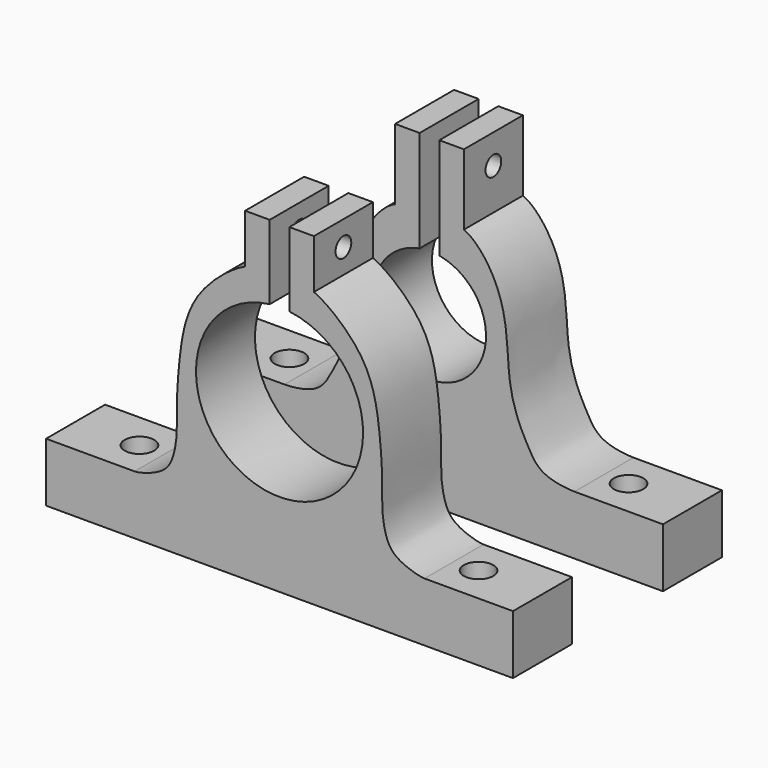
from build123d import *

# Parameters (mm, degrees)
F1_DEPTH  = 15
F3_W      = 4
F3_H      = 15
F4_DEPTH  = 25
F5_R      = 3
F6_DEPTH  = 25
F7_R      = 2
F8_DEPTH  = 25
F10_DEPTH = 15
F11_R     = 3
F12_DEPTH = 25
F13_W     = 4
F13_H     = 15
F14_DEPTH = 25
F15_R     = 2
F16_DEPTH = 25


# Not quite as in the source:
# - a feature names something its author has since deleted; it is built from what else it names


with BuildPart() as f1:
    # F0 (on Front) → F1 (new body)
    with BuildSketch(Plane.XZ):
        with BuildLine():
            Line((-125.6711477041, 86.9706617594), (-125.6711477041, 107.4706617594))
            Line((-125.6711477041, 107.4706617594), (-132.6711477041, 107.4706617594))
            Line((-132.6711477041, 107.4706617594), (-132.6711477041, 93.0804520496))
            add(Edge.make_bspline(
                [(-132.6711477041, 93.0804520496), (-134.8444351683, 92.1647803788), (-139.3318293406, 86.8815258397), (-141.6489540104, 77.9315652386), (-141.6385080687, 68.53125191), (-143.7808164235, 62.0408932683), (-145.6725641316, 58.6368592184), (-148.1505873732, 53.9411069546), (-153.9757510035, 53.4706617594), (-155.1711477041, 53.4706617594)],
                knots=[0, 0, 0, 0, 0.1589153696, 0.3266349591, 0.4941602985, 0.6338202377, 0.7405177517, 0.8628095578, 1, 1, 1, 1], degree=3))
            Line((-155.1711477041, 53.4706617594), (-173.1711477041, 53.4706617594))
            Line((-173.1711477041, 53.4706617594), (-173.1711477041, 41.4706617594))
            Line((-173.1711477041, 41.4706617594), (-125.6711477041, 41.4706617594))
            Line((-125.6711477041, 41.4706617594), (-125.6711477041, 63.9706617594))
            ThreePointArc((-125.6711477041, 63.9706617594), (-137.1711477041, 75.4706617594), (-125.6711477041, 86.9706617594))
        make_face()
        with BuildLine():
            Line((-118.6711477041, 107.4706617594), (-125.6711477041, 107.4706617594))
            Line((-125.6711477041, 107.4706617594), (-125.6711477041, 86.9706617594))
            ThreePointArc((-125.6711477041, 86.9706617594), (-114.1711477041, 75.4706617594), (-125.6711477041, 63.9706617594))
            Line((-125.6711477041, 63.9706617594), (-125.6711477041, 41.4706617594))
            Line((-125.6711477041, 41.4706617594), (-78.1711477041, 41.4706617594))
            Line((-78.1711477041, 41.4706617594), (-78.1711477041, 53.4706617594))
            Line((-78.1711477041, 53.4706617594), (-96.1711477041, 53.4706617594))
            add(Edge.make_bspline(
                [(-118.6711477041, 93.0804520496), (-116.49786024, 92.1647803788), (-112.0104660676, 86.8815258397), (-109.6933413979, 77.9315652386), (-109.7037873395, 68.53125191), (-107.5614789847, 62.0408932683), (-105.6697312766, 58.6368592184), (-103.191708035, 53.9411069546), (-97.3665444048, 53.4706617594), (-96.1711477041, 53.4706617594)],
                knots=[0, 0, 0, 0, 0.1589153696, 0.3266349591, 0.4941602985, 0.6338202377, 0.7405177517, 0.8628095578, 1, 1, 1, 1], degree=3))
            Line((-118.6711477041, 93.0804520496), (-118.6711477041, 107.4706617594))
        make_face()
    extrude(amount=F1_DEPTH)

    # F3 (on face) → F4 (cut)
    with BuildSketch(Plane.XY.offset(107.4706617594)):
        with Locations((-125.6711477041, -7.5)):
            Rectangle(F3_W, F3_H)
    extrude(amount=-F4_DEPTH, mode=Mode.SUBTRACT)

    # F5 (on face) → F6 (cut)
    with BuildSketch(Plane(origin=(0, 0, 41.4706617594), x_dir=(1, 0, 0), z_dir=(0, 0, -1))):
        with Locations((-160.1711477041, 7.5)):
            Circle(F5_R)
        with Locations((-91.1711477041, 7.5)):
            Circle(F5_R)
    extrude(amount=-F6_DEPTH, mode=Mode.SUBTRACT)

    # F7 (on face) → F8 (cut)
    with BuildSketch(Plane(origin=(-132.6711477041, 0, 0), x_dir=(0, -1, 0), z_dir=(-1, 0, 0))):
        with Locations((7.5, 101.4706617594)):
            Circle(F7_R)
    extrude(amount=-F8_DEPTH, mode=Mode.SUBTRACT)


with BuildPart() as f10:
    # F9 (on offset) → F10 (new body)
    with BuildSketch(Plane.XZ.offset(38)):
        with BuildLine():
            Line((-125.7859611511, 92.3226373494), (-125.7859611511, 107.3226373494))
            Line((-125.7859611511, 107.3226373494), (-132.7859611511, 107.3226373494))
            Line((-132.7859611511, 107.3226373494), (-132.7859611511, 97.3226373494))
            add(Edge.make_bspline(
                [(-132.7859611511, 97.3226373494), (-135.3544034247, 96.2404750185), (-144.1033534904, 89.486584983), (-146.1690728794, 77.6369899314), (-146.7872760168, 68.4366512578), (-146.5336940779, 62.8295997289), (-147.3177284091, 58.2938754382), (-149.1347203045, 54.8107556411), (-154.1745465523, 53.3226373494), (-155.2859611511, 53.3226373494)],
                knots=[0, 0, 0, 0, 0.1878099238, 0.3732226175, 0.5329240866, 0.6574575834, 0.7678477858, 0.8724478156, 1, 1, 1, 1], degree=3))
            Line((-155.2859611511, 53.3226373494), (-173.2859611511, 53.3226373494))
            Line((-173.2859611511, 53.3226373494), (-173.2859611511, 41.3226373494))
            Line((-173.2859611511, 41.3226373494), (-125.7859611511, 41.3226373494))
            Line((-125.7859611511, 41.3226373494), (-125.7859611511, 58.3226373494))
            ThreePointArc((-125.7859611511, 58.3226373494), (-142.7859611511, 75.3226373494), (-125.7859611511, 92.3226373494))
        make_face()
        with BuildLine():
            Line((-118.7859611511, 107.3226373494), (-125.7859611511, 107.3226373494))
            Line((-125.7859611511, 107.3226373494), (-125.7859611511, 92.3226373494))
            ThreePointArc((-125.7859611511, 92.3226373494), (-108.7859611511, 75.3226373494), (-125.7859611511, 58.3226373494))
            Line((-125.7859611511, 58.3226373494), (-125.7859611511, 41.3226373494))
            Line((-125.7859611511, 41.3226373494), (-78.2859611511, 41.3226373494))
            Line((-78.2859611511, 41.3226373494), (-78.2859611511, 53.3226373494))
            Line((-78.2859611511, 53.3226373494), (-96.2859611511, 53.3226373494))
            add(Edge.make_bspline(
                [(-118.7859611511, 97.3226373494), (-116.2175188776, 96.2404750185), (-107.4685688118, 89.486584983), (-105.4028494228, 77.6369899314), (-104.7846462854, 68.4366512578), (-105.0382282244, 62.8295997289), (-104.2541938932, 58.2938754382), (-102.4372019978, 54.8107556411), (-97.39737575, 53.3226373494), (-96.2859611511, 53.3226373494)],
                knots=[0, 0, 0, 0, 0.1878099238, 0.3732226175, 0.5329240866, 0.6574575834, 0.7678477858, 0.8724478156, 1, 1, 1, 1], degree=3))
            Line((-118.7859611511, 97.3226373494), (-118.7859611511, 107.3226373494))
        make_face()
    extrude(amount=F10_DEPTH)

    # F11 (on face) → F12 (cut)
    with BuildSketch(Plane(origin=(0, 0, 41.3226373494), x_dir=(1, 0, 0), z_dir=(0, 0, -1))):
        with Locations((-160.2859611511, 45.5)):
            Circle(F11_R)
        with Locations((-91.2859611511, 45.5)):
            Circle(F11_R)
    extrude(amount=-F12_DEPTH, mode=Mode.SUBTRACT)

    # F13 (on face) → F14 (cut)
    with BuildSketch(Plane.XY.offset(107.3226373494)):
        with Locations((-125.7859611511, -45.5)):
            Rectangle(F13_W, F13_H)
    extrude(amount=-F14_DEPTH, mode=Mode.SUBTRACT)

    # F15 (on face) → F16 (cut)
    with BuildSketch(Plane.YZ.offset(-118.7859611511)):
        with Locations((-45.5, 102.3226373494)):
            Circle(F15_R)
    extrude(amount=-F16_DEPTH, mode=Mode.SUBTRACT)


solid = Compound([f1.part, f10.part])
